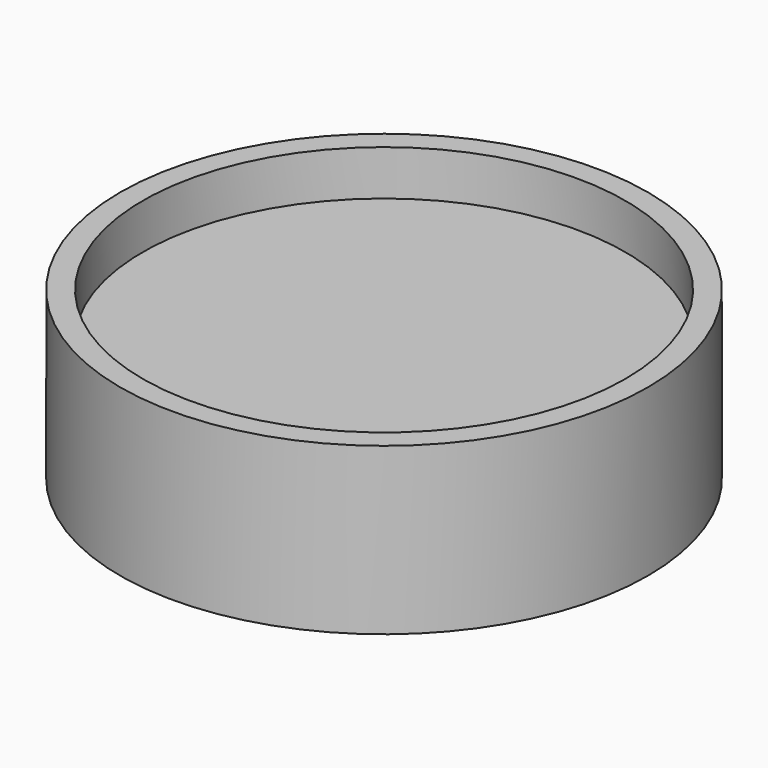
from build123d import *

# Parameters (mm, degrees)
F0_R     = 17.5
F1_DEPTH = 11
F2_R     = 16
F3_DEPTH = 3
F4_W     = 13.5
F4_H     = 1.7
F5_DEPTH = 5


with BuildPart() as f1:
    # F0 (on Top) → F1 (new body)
    with BuildSketch(Plane.XY):
        Circle(F0_R)
    extrude(amount=F1_DEPTH)

    # F2 (on face) → F3 (cut)
    with BuildSketch(Plane.XY.offset(11)):
        Circle(F2_R)
    extrude(amount=-F3_DEPTH, mode=Mode.SUBTRACT)

    # F4 (on face) → F5 (cut)
    with BuildSketch(Plane(origin=(0, 0, 0), x_dir=(1, 0, 0), z_dir=(0, 0, -1))):
        with BuildLine():
            Line((-1.7, -17.4172328457), (-1.7, -1.7))
            Line((-1.7, -1.7), (-5.1, -1.7))
            Line((-5.1, -1.7), (-5.1, -16.7403703663))
            ThreePointArc((-5.1, -16.7403703663), (-3.4168019703, -17.1632008756), (-1.7, -17.4172328457))
        make_face()
        Polygon((0, -1.7), (0, 0), (-13.5, 0), (-13.5, -1.7), (-5.1, -1.7), (-1.7, -1.7), align=None)
        Polygon((13.5, 0), (0, 0), (0, -1.7), (1.7, -1.7), (13.5, -1.7), align=None)
        with Locations((6.75, 0.85)):
            Rectangle(F4_W, F4_H)
        with Locations((-6.75, 0.85)):
            Rectangle(F4_W, F4_H)
    extrude(amount=-F5_DEPTH, mode=Mode.SUBTRACT)


solid = f1.part
